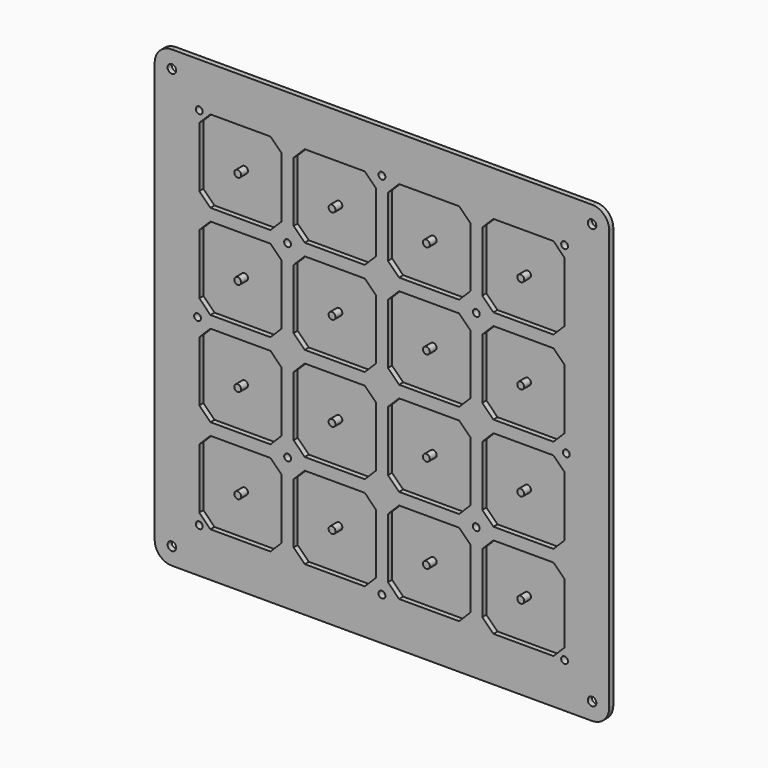
from build123d import *

# Parameters (mm, degrees)
F1_DEPTH      = 12
F2_START      = -12
F0_R          = 2
F2_DEPTH      = 6
F3_DEPTH      = 6
F4_DEPTH      = 20
F4_DEPTH_BACK = 5
F5_R          = 2.5
F6_DEPTH      = 3
F7_SIZE       = 2
F8_D          = 4
F8_2_D        = 4
F9_D          = 4


with BuildPart() as f1:
    # F0 (on Front) → F1 (new body)
    with BuildSketch(Plane.XZ):
        with BuildLine():
            Line((106.5, 111.5), (-106.5, 111.5))
            ThreePointArc((-106.5, 111.5), (-110.0355339059, 110.0355339059), (-111.5, 106.5))
            Line((-111.5, 106.5), (-111.5, -106.5))
            ThreePointArc((-111.5, -106.5), (-110.0355339059, -110.0355339059), (-106.5, -111.5))
            Line((-106.5, -111.5), (106.5, -111.5))
            ThreePointArc((106.5, -111.5), (110.0355339059, -110.0355339059), (111.5, -106.5))
            Line((111.5, -106.5), (111.5, 106.5))
            ThreePointArc((111.5, 106.5), (110.0355339059, 110.0355339059), (106.5, 111.5))
        make_face()
        Polygon((-64.5710678119, -57.5), (-57.5, -64.5710678119), (-57.5, -82.5), (-57.5, -100.4289321881), (-64.5710678119, -107.5), (-82.5, -107.5), (-100.4289321881, -107.5), (-107.5, -100.4289321881), (-107.5, -82.5), (-107.5, -64.5710678119), (-100.4289321881, -57.5), (-82.5, -57.5), align=None, mode=Mode.SUBTRACT)
        Polygon((-9.5710678119, -57.5), (-2.5, -64.5710678119), (-2.5, -82.5), (-2.5, -100.4289321881), (-9.5710678119, -107.5), (-27.5, -107.5), (-45.4289321881, -107.5), (-52.5, -100.4289321881), (-52.5, -82.5), (-52.5, -64.5710678119), (-45.4289321881, -57.5), (-27.5, -57.5), align=None, mode=Mode.SUBTRACT)
        Polygon((-64.5710678119, -2.5), (-57.5, -9.5710678119), (-57.5, -27.5), (-57.5, -45.4289321881), (-64.5710678119, -52.5), (-82.5, -52.5), (-100.4289321881, -52.5), (-107.5, -45.4289321881), (-107.5, -27.5), (-107.5, -9.5710678119), (-100.4289321881, -2.5), (-82.5, -2.5), align=None, mode=Mode.SUBTRACT)
        Polygon((-9.5710678119, -2.5), (-2.5, -9.5710678119), (-2.5, -27.5), (-2.5, -45.4289321881), (-9.5710678119, -52.5), (-27.5, -52.5), (-45.4289321881, -52.5), (-52.5, -45.4289321881), (-52.5, -27.5), (-52.5, -9.5710678119), (-45.4289321881, -2.5), (-27.5, -2.5), align=None, mode=Mode.SUBTRACT)
        Polygon((45.4289321881, -57.5), (52.5, -64.5710678119), (52.5, -82.5), (52.5, -100.4289321881), (45.4289321881, -107.5), (27.5, -107.5), (9.5710678119, -107.5), (2.5, -100.4289321881), (2.5, -82.5), (2.5, -64.5710678119), (9.5710678119, -57.5), (27.5, -57.5), align=None, mode=Mode.SUBTRACT)
        Polygon((100.4289321881, -57.5), (107.5, -64.5710678119), (107.5, -82.5), (107.5, -100.4289321881), (100.4289321881, -107.5), (82.5, -107.5), (64.5710678119, -107.5), (57.5, -100.4289321881), (57.5, -82.5), (57.5, -64.5710678119), (64.5710678119, -57.5), (82.5, -57.5), align=None, mode=Mode.SUBTRACT)
        Polygon((45.4289321881, -2.5), (52.5, -9.5710678119), (52.5, -27.5), (52.5, -45.4289321881), (45.4289321881, -52.5), (27.5, -52.5), (9.5710678119, -52.5), (2.5, -45.4289321881), (2.5, -27.5), (2.5, -9.5710678119), (9.5710678119, -2.5), (27.5, -2.5), align=None, mode=Mode.SUBTRACT)
        Polygon((100.4289321881, -2.5), (107.5, -9.5710678119), (107.5, -27.5), (107.5, -45.4289321881), (100.4289321881, -52.5), (82.5, -52.5), (64.5710678119, -52.5), (57.5, -45.4289321881), (57.5, -27.5), (57.5, -9.5710678119), (64.5710678119, -2.5), (82.5, -2.5), align=None, mode=Mode.SUBTRACT)
        Polygon((-64.5710678119, 52.5), (-57.5, 45.4289321881), (-57.5, 27.5), (-57.5, 9.5710678119), (-64.5710678119, 2.5), (-82.5, 2.5), (-100.4289321881, 2.5), (-107.5, 9.5710678119), (-107.5, 27.5), (-107.5, 45.4289321881), (-100.4289321881, 52.5), (-82.5, 52.5), align=None, mode=Mode.SUBTRACT)
        Polygon((-9.5710678119, 52.5), (-2.5, 45.4289321881), (-2.5, 27.5), (-2.5, 9.5710678119), (-9.5710678119, 2.5), (-27.5, 2.5), (-45.4289321881, 2.5), (-52.5, 9.5710678119), (-52.5, 27.5), (-52.5, 45.4289321881), (-45.4289321881, 52.5), (-27.5, 52.5), align=None, mode=Mode.SUBTRACT)
        Polygon((-107.5, 64.5710678119), (-107.5, 82.5), (-107.5, 100.4289321881), (-100.4289321881, 107.5), (-82.5, 107.5), (-64.5710678119, 107.5), (-57.5, 100.4289321881), (-57.5, 82.5), (-57.5, 64.5710678119), (-64.5710678119, 57.5), (-82.5, 57.5), (-100.4289321881, 57.5), align=None, mode=Mode.SUBTRACT)
        Polygon((-9.5710678119, 107.5), (-2.5, 100.4289321881), (-2.5, 82.5), (-2.5, 64.5710678119), (-9.5710678119, 57.5), (-27.5, 57.5), (-45.4289321881, 57.5), (-52.5, 64.5710678119), (-52.5, 82.5), (-52.5, 100.4289321881), (-45.4289321881, 107.5), (-27.5, 107.5), align=None, mode=Mode.SUBTRACT)
        Polygon((45.4289321881, 52.5), (52.5, 45.4289321881), (52.5, 27.5), (52.5, 9.5710678119), (45.4289321881, 2.5), (27.5, 2.5), (9.5710678119, 2.5), (2.5, 9.5710678119), (2.5, 27.5), (2.5, 45.4289321881), (9.5710678119, 52.5), (27.5, 52.5), align=None, mode=Mode.SUBTRACT)
        Polygon((100.4289321881, 52.5), (107.5, 45.4289321881), (107.5, 27.5), (107.5, 9.5710678119), (100.4289321881, 2.5), (82.5, 2.5), (64.5710678119, 2.5), (57.5, 9.5710678119), (57.5, 27.5), (57.5, 45.4289321881), (64.5710678119, 52.5), (82.5, 52.5), align=None, mode=Mode.SUBTRACT)
        Polygon((45.4289321881, 107.5), (52.5, 100.4289321881), (52.5, 82.5), (52.5, 64.5710678119), (45.4289321881, 57.5), (27.5, 57.5), (9.5710678119, 57.5), (2.5, 64.5710678119), (2.5, 82.5), (2.5, 100.4289321881), (9.5710678119, 107.5), (27.5, 107.5), align=None, mode=Mode.SUBTRACT)
        Polygon((100.4289321881, 107.5), (107.5, 100.4289321881), (107.5, 82.5), (107.5, 64.5710678119), (100.4289321881, 57.5), (82.5, 57.5), (64.5710678119, 57.5), (57.5, 64.5710678119), (57.5, 82.5), (57.5, 100.4289321881), (64.5710678119, 107.5), (82.5, 107.5), align=None, mode=Mode.SUBTRACT)
    extrude(amount=-F1_DEPTH)

    # F8 (through all)
    with Locations(Plane.XZ):
        with Locations((106.5, 106.5), (0, 107.5), (-106.5, 106.5), (-107.5, 0), (107.5, 0), (106.5, -106.5), (0, -107.5), (-106.5, -106.5), (-55, 55), (55, 55), (55, -55), (-55, -55)):
            Hole(F8_D / 2)


with BuildPart() as f2:
    # F0 (on Front) → F2 (new body)
    with BuildSketch(Plane.XZ.offset(F2_START)):
        with BuildLine():
            Line((106.5, 111.5), (-106.5, 111.5))
            ThreePointArc((-106.5, 111.5), (-110.0355339059, 110.0355339059), (-111.5, 106.5))
            Line((-111.5, 106.5), (-111.5, -106.5))
            ThreePointArc((-111.5, -106.5), (-110.0355339059, -110.0355339059), (-106.5, -111.5))
            Line((-106.5, -111.5), (106.5, -111.5))
            ThreePointArc((106.5, -111.5), (110.0355339059, -110.0355339059), (111.5, -106.5))
            Line((111.5, -106.5), (111.5, 106.5))
            ThreePointArc((111.5, 106.5), (110.0355339059, 110.0355339059), (106.5, 111.5))
        make_face()
        Polygon((-64.5710678119, -57.5), (-57.5, -64.5710678119), (-57.5, -82.5), (-57.5, -100.4289321881), (-64.5710678119, -107.5), (-82.5, -107.5), (-100.4289321881, -107.5), (-107.5, -100.4289321881), (-107.5, -82.5), (-107.5, -64.5710678119), (-100.4289321881, -57.5), (-82.5, -57.5), align=None, mode=Mode.SUBTRACT)
        Polygon((-9.5710678119, -57.5), (-2.5, -64.5710678119), (-2.5, -82.5), (-2.5, -100.4289321881), (-9.5710678119, -107.5), (-27.5, -107.5), (-45.4289321881, -107.5), (-52.5, -100.4289321881), (-52.5, -82.5), (-52.5, -64.5710678119), (-45.4289321881, -57.5), (-27.5, -57.5), align=None, mode=Mode.SUBTRACT)
        Polygon((-64.5710678119, -2.5), (-57.5, -9.5710678119), (-57.5, -27.5), (-57.5, -45.4289321881), (-64.5710678119, -52.5), (-82.5, -52.5), (-100.4289321881, -52.5), (-107.5, -45.4289321881), (-107.5, -27.5), (-107.5, -9.5710678119), (-100.4289321881, -2.5), (-82.5, -2.5), align=None, mode=Mode.SUBTRACT)
        Polygon((-9.5710678119, -2.5), (-2.5, -9.5710678119), (-2.5, -27.5), (-2.5, -45.4289321881), (-9.5710678119, -52.5), (-27.5, -52.5), (-45.4289321881, -52.5), (-52.5, -45.4289321881), (-52.5, -27.5), (-52.5, -9.5710678119), (-45.4289321881, -2.5), (-27.5, -2.5), align=None, mode=Mode.SUBTRACT)
        Polygon((45.4289321881, -57.5), (52.5, -64.5710678119), (52.5, -82.5), (52.5, -100.4289321881), (45.4289321881, -107.5), (27.5, -107.5), (9.5710678119, -107.5), (2.5, -100.4289321881), (2.5, -82.5), (2.5, -64.5710678119), (9.5710678119, -57.5), (27.5, -57.5), align=None, mode=Mode.SUBTRACT)
        Polygon((100.4289321881, -57.5), (107.5, -64.5710678119), (107.5, -82.5), (107.5, -100.4289321881), (100.4289321881, -107.5), (82.5, -107.5), (64.5710678119, -107.5), (57.5, -100.4289321881), (57.5, -82.5), (57.5, -64.5710678119), (64.5710678119, -57.5), (82.5, -57.5), align=None, mode=Mode.SUBTRACT)
        Polygon((45.4289321881, -2.5), (52.5, -9.5710678119), (52.5, -27.5), (52.5, -45.4289321881), (45.4289321881, -52.5), (27.5, -52.5), (9.5710678119, -52.5), (2.5, -45.4289321881), (2.5, -27.5), (2.5, -9.5710678119), (9.5710678119, -2.5), (27.5, -2.5), align=None, mode=Mode.SUBTRACT)
        Polygon((100.4289321881, -2.5), (107.5, -9.5710678119), (107.5, -27.5), (107.5, -45.4289321881), (100.4289321881, -52.5), (82.5, -52.5), (64.5710678119, -52.5), (57.5, -45.4289321881), (57.5, -27.5), (57.5, -9.5710678119), (64.5710678119, -2.5), (82.5, -2.5), align=None, mode=Mode.SUBTRACT)
        Polygon((-64.5710678119, 52.5), (-57.5, 45.4289321881), (-57.5, 27.5), (-57.5, 9.5710678119), (-64.5710678119, 2.5), (-82.5, 2.5), (-100.4289321881, 2.5), (-107.5, 9.5710678119), (-107.5, 27.5), (-107.5, 45.4289321881), (-100.4289321881, 52.5), (-82.5, 52.5), align=None, mode=Mode.SUBTRACT)
        Polygon((-9.5710678119, 52.5), (-2.5, 45.4289321881), (-2.5, 27.5), (-2.5, 9.5710678119), (-9.5710678119, 2.5), (-27.5, 2.5), (-45.4289321881, 2.5), (-52.5, 9.5710678119), (-52.5, 27.5), (-52.5, 45.4289321881), (-45.4289321881, 52.5), (-27.5, 52.5), align=None, mode=Mode.SUBTRACT)
        Polygon((-107.5, 64.5710678119), (-107.5, 82.5), (-107.5, 100.4289321881), (-100.4289321881, 107.5), (-82.5, 107.5), (-64.5710678119, 107.5), (-57.5, 100.4289321881), (-57.5, 82.5), (-57.5, 64.5710678119), (-64.5710678119, 57.5), (-82.5, 57.5), (-100.4289321881, 57.5), align=None, mode=Mode.SUBTRACT)
        Polygon((-9.5710678119, 107.5), (-2.5, 100.4289321881), (-2.5, 82.5), (-2.5, 64.5710678119), (-9.5710678119, 57.5), (-27.5, 57.5), (-45.4289321881, 57.5), (-52.5, 64.5710678119), (-52.5, 82.5), (-52.5, 100.4289321881), (-45.4289321881, 107.5), (-27.5, 107.5), align=None, mode=Mode.SUBTRACT)
        Polygon((45.4289321881, 52.5), (52.5, 45.4289321881), (52.5, 27.5), (52.5, 9.5710678119), (45.4289321881, 2.5), (27.5, 2.5), (9.5710678119, 2.5), (2.5, 9.5710678119), (2.5, 27.5), (2.5, 45.4289321881), (9.5710678119, 52.5), (27.5, 52.5), align=None, mode=Mode.SUBTRACT)
        Polygon((100.4289321881, 52.5), (107.5, 45.4289321881), (107.5, 27.5), (107.5, 9.5710678119), (100.4289321881, 2.5), (82.5, 2.5), (64.5710678119, 2.5), (57.5, 9.5710678119), (57.5, 27.5), (57.5, 45.4289321881), (64.5710678119, 52.5), (82.5, 52.5), align=None, mode=Mode.SUBTRACT)
        Polygon((45.4289321881, 107.5), (52.5, 100.4289321881), (52.5, 82.5), (52.5, 64.5710678119), (45.4289321881, 57.5), (27.5, 57.5), (9.5710678119, 57.5), (2.5, 64.5710678119), (2.5, 82.5), (2.5, 100.4289321881), (9.5710678119, 107.5), (27.5, 107.5), align=None, mode=Mode.SUBTRACT)
        Polygon((100.4289321881, 107.5), (107.5, 100.4289321881), (107.5, 82.5), (107.5, 64.5710678119), (100.4289321881, 57.5), (82.5, 57.5), (64.5710678119, 57.5), (57.5, 64.5710678119), (57.5, 82.5), (57.5, 100.4289321881), (64.5710678119, 107.5), (82.5, 107.5), align=None, mode=Mode.SUBTRACT)
        Polygon((107.5, -82.5), (107.5, -64.5710678119), (100.4289321881, -57.5), (82.5, -57.5), (64.5710678119, -57.5), (57.5, -64.5710678119), (57.5, -82.5), (57.5, -100.4289321881), (64.5710678119, -107.5), (82.5, -107.5), (100.4289321881, -107.5), (107.5, -100.4289321881), align=None)
        with Locations((82.5, -82.5)):
            Circle(F0_R, mode=Mode.SUBTRACT)
        Polygon((52.5, -82.5), (52.5, -64.5710678119), (45.4289321881, -57.5), (27.5, -57.5), (9.5710678119, -57.5), (2.5, -64.5710678119), (2.5, -82.5), (2.5, -100.4289321881), (9.5710678119, -107.5), (27.5, -107.5), (45.4289321881, -107.5), (52.5, -100.4289321881), align=None)
        with Locations((27.5, -82.5)):
            Circle(F0_R, mode=Mode.SUBTRACT)
        Polygon((-2.5, -82.5), (-2.5, -64.5710678119), (-9.5710678119, -57.5), (-27.5, -57.5), (-45.4289321881, -57.5), (-52.5, -64.5710678119), (-52.5, -82.5), (-52.5, -100.4289321881), (-45.4289321881, -107.5), (-27.5, -107.5), (-9.5710678119, -107.5), (-2.5, -100.4289321881), align=None)
        with Locations((-27.5, -82.5)):
            Circle(F0_R, mode=Mode.SUBTRACT)
        Polygon((-57.5, -82.5), (-57.5, -64.5710678119), (-64.5710678119, -57.5), (-82.5, -57.5), (-100.4289321881, -57.5), (-107.5, -64.5710678119), (-107.5, -82.5), (-107.5, -100.4289321881), (-100.4289321881, -107.5), (-82.5, -107.5), (-64.5710678119, -107.5), (-57.5, -100.4289321881), align=None)
        with Locations((-82.5, -82.5)):
            Circle(F0_R, mode=Mode.SUBTRACT)
        Polygon((-2.5, -27.5), (-2.5, -9.5710678119), (-9.5710678119, -2.5), (-27.5, -2.5), (-45.4289321881, -2.5), (-52.5, -9.5710678119), (-52.5, -27.5), (-52.5, -45.4289321881), (-45.4289321881, -52.5), (-27.5, -52.5), (-9.5710678119, -52.5), (-2.5, -45.4289321881), align=None)
        with Locations((-27.5, -27.5)):
            Circle(F0_R, mode=Mode.SUBTRACT)
        Polygon((-57.5, -27.5), (-57.5, -9.5710678119), (-64.5710678119, -2.5), (-82.5, -2.5), (-100.4289321881, -2.5), (-107.5, -9.5710678119), (-107.5, -27.5), (-107.5, -45.4289321881), (-100.4289321881, -52.5), (-82.5, -52.5), (-64.5710678119, -52.5), (-57.5, -45.4289321881), align=None)
        with Locations((-82.5, -27.5)):
            Circle(F0_R, mode=Mode.SUBTRACT)
        Polygon((52.5, -27.5), (52.5, -9.5710678119), (45.4289321881, -2.5), (27.5, -2.5), (9.5710678119, -2.5), (2.5, -9.5710678119), (2.5, -27.5), (2.5, -45.4289321881), (9.5710678119, -52.5), (27.5, -52.5), (45.4289321881, -52.5), (52.5, -45.4289321881), align=None)
        with Locations((27.5, -27.5)):
            Circle(F0_R, mode=Mode.SUBTRACT)
        Polygon((107.5, -27.5), (107.5, -9.5710678119), (100.4289321881, -2.5), (82.5, -2.5), (64.5710678119, -2.5), (57.5, -9.5710678119), (57.5, -27.5), (57.5, -45.4289321881), (64.5710678119, -52.5), (82.5, -52.5), (100.4289321881, -52.5), (107.5, -45.4289321881), align=None)
        with Locations((82.5, -27.5)):
            Circle(F0_R, mode=Mode.SUBTRACT)
        Polygon((107.5, 27.5), (107.5, 45.4289321881), (100.4289321881, 52.5), (82.5, 52.5), (64.5710678119, 52.5), (57.5, 45.4289321881), (57.5, 27.5), (57.5, 9.5710678119), (64.5710678119, 2.5), (82.5, 2.5), (100.4289321881, 2.5), (107.5, 9.5710678119), align=None)
        with Locations((82.5, 27.5)):
            Circle(F0_R, mode=Mode.SUBTRACT)
        Polygon((52.5, 27.5), (52.5, 45.4289321881), (45.4289321881, 52.5), (27.5, 52.5), (9.5710678119, 52.5), (2.5, 45.4289321881), (2.5, 27.5), (2.5, 9.5710678119), (9.5710678119, 2.5), (27.5, 2.5), (45.4289321881, 2.5), (52.5, 9.5710678119), align=None)
        with Locations((27.5, 27.5)):
            Circle(F0_R, mode=Mode.SUBTRACT)
        Polygon((-2.5, 27.5), (-2.5, 45.4289321881), (-9.5710678119, 52.5), (-27.5, 52.5), (-45.4289321881, 52.5), (-52.5, 45.4289321881), (-52.5, 27.5), (-52.5, 9.5710678119), (-45.4289321881, 2.5), (-27.5, 2.5), (-9.5710678119, 2.5), (-2.5, 9.5710678119), align=None)
        with Locations((-27.5, 27.5)):
            Circle(F0_R, mode=Mode.SUBTRACT)
        Polygon((-57.5, 27.5), (-57.5, 45.4289321881), (-64.5710678119, 52.5), (-82.5, 52.5), (-100.4289321881, 52.5), (-107.5, 45.4289321881), (-107.5, 27.5), (-107.5, 9.5710678119), (-100.4289321881, 2.5), (-82.5, 2.5), (-64.5710678119, 2.5), (-57.5, 9.5710678119), align=None)
        with Locations((-82.5, 27.5)):
            Circle(F0_R, mode=Mode.SUBTRACT)
        Polygon((-107.5, 100.4289321881), (-107.5, 82.5), (-107.5, 64.5710678119), (-100.4289321881, 57.5), (-82.5, 57.5), (-64.5710678119, 57.5), (-57.5, 64.5710678119), (-57.5, 82.5), (-57.5, 100.4289321881), (-64.5710678119, 107.5), (-82.5, 107.5), (-100.4289321881, 107.5), align=None)
        with Locations((-82.5, 82.5)):
            Circle(F0_R, mode=Mode.SUBTRACT)
        Polygon((-2.5, 82.5), (-2.5, 100.4289321881), (-9.5710678119, 107.5), (-27.5, 107.5), (-45.4289321881, 107.5), (-52.5, 100.4289321881), (-52.5, 82.5), (-52.5, 64.5710678119), (-45.4289321881, 57.5), (-27.5, 57.5), (-9.5710678119, 57.5), (-2.5, 64.5710678119), align=None)
        with Locations((-27.5, 82.5)):
            Circle(F0_R, mode=Mode.SUBTRACT)
        Polygon((52.5, 82.5), (52.5, 100.4289321881), (45.4289321881, 107.5), (27.5, 107.5), (9.5710678119, 107.5), (2.5, 100.4289321881), (2.5, 82.5), (2.5, 64.5710678119), (9.5710678119, 57.5), (27.5, 57.5), (45.4289321881, 57.5), (52.5, 64.5710678119), align=None)
        with Locations((27.5, 82.5)):
            Circle(F0_R, mode=Mode.SUBTRACT)
        Polygon((107.5, 82.5), (107.5, 100.4289321881), (100.4289321881, 107.5), (82.5, 107.5), (64.5710678119, 107.5), (57.5, 100.4289321881), (57.5, 82.5), (57.5, 64.5710678119), (64.5710678119, 57.5), (82.5, 57.5), (100.4289321881, 57.5), (107.5, 64.5710678119), align=None)
        with Locations((82.5, 82.5)):
            Circle(F0_R, mode=Mode.SUBTRACT)
    extrude(amount=-F2_DEPTH)

    # F7
    f7_edges = [f2.edges().sort_by_distance(p)[0] for p in [
        (-84.5, 12, 82.5),
        (-29.5, 12, 82.5),
        (25.5, 12, 82.5),
        (80.5, 12, 82.5),
        (80.5, 12, 27.5),
        (25.5, 12, 27.5),
        (-29.5, 12, 27.5),
        (-84.5, 12, 27.5),
        (-84.5, 12, -27.5),
        (-29.5, 12, -27.5),
        (25.5, 12, -27.5),
        (80.5, 12, -27.5),
        (80.5, 12, -82.5),
        (25.5, 12, -82.5),
        (-29.5, 12, -82.5),
        (-84.5, 12, -82.5),
    ]]
    chamfer(f7_edges, length=F7_SIZE)

    # F8#2 (through all)
    with Locations(Plane.XZ):
        with Locations((106.5, 106.5), (0, 107.5), (-106.5, 106.5), (-107.5, 0), (107.5, 0), (106.5, -106.5), (0, -107.5), (-106.5, -106.5), (-55, 55), (55, 55), (55, -55), (-55, -55)):
            Hole(F8_2_D / 2)


with BuildPart() as f3:
    # F0 (on Front) → F3 (new body)
    with BuildSketch(Plane.XZ):
        Polygon((-107.5, 100.4289321881), (-107.5, 82.5), (-107.5, 64.5710678119), (-100.4289321881, 57.5), (-82.5, 57.5), (-64.5710678119, 57.5), (-57.5, 64.5710678119), (-57.5, 82.5), (-57.5, 100.4289321881), (-64.5710678119, 107.5), (-82.5, 107.5), (-100.4289321881, 107.5), align=None)
        with Locations((-82.5, 82.5)):
            Circle(F0_R, mode=Mode.SUBTRACT)
    extrude(amount=-F3_DEPTH)


with BuildPart() as f3b:
    # F0 (on Front) → F3, piece 2 (new body)
    with BuildSketch(Plane.XZ):
        Polygon((-2.5, 82.5), (-2.5, 100.4289321881), (-9.5710678119, 107.5), (-27.5, 107.5), (-45.4289321881, 107.5), (-52.5, 100.4289321881), (-52.5, 82.5), (-52.5, 64.5710678119), (-45.4289321881, 57.5), (-27.5, 57.5), (-9.5710678119, 57.5), (-2.5, 64.5710678119), align=None)
        with Locations((-27.5, 82.5)):
            Circle(F0_R, mode=Mode.SUBTRACT)
    extrude(amount=-F3_DEPTH)


with BuildPart() as f3c:
    # F0 (on Front) → F3, piece 3 (new body)
    with BuildSketch(Plane.XZ):
        Polygon((52.5, 82.5), (52.5, 100.4289321881), (45.4289321881, 107.5), (27.5, 107.5), (9.5710678119, 107.5), (2.5, 100.4289321881), (2.5, 82.5), (2.5, 64.5710678119), (9.5710678119, 57.5), (27.5, 57.5), (45.4289321881, 57.5), (52.5, 64.5710678119), align=None)
        with Locations((27.5, 82.5)):
            Circle(F0_R, mode=Mode.SUBTRACT)
    extrude(amount=-F3_DEPTH)


with BuildPart() as f3d:
    # F0 (on Front) → F3, piece 4 (new body)
    with BuildSketch(Plane.XZ):
        Polygon((107.5, 82.5), (107.5, 100.4289321881), (100.4289321881, 107.5), (82.5, 107.5), (64.5710678119, 107.5), (57.5, 100.4289321881), (57.5, 82.5), (57.5, 64.5710678119), (64.5710678119, 57.5), (82.5, 57.5), (100.4289321881, 57.5), (107.5, 64.5710678119), align=None)
        with Locations((82.5, 82.5)):
            Circle(F0_R, mode=Mode.SUBTRACT)
    extrude(amount=-F3_DEPTH)


with BuildPart() as f3e:
    # F0 (on Front) → F3, piece 5 (new body)
    with BuildSketch(Plane.XZ):
        Polygon((-57.5, 27.5), (-57.5, 45.4289321881), (-64.5710678119, 52.5), (-82.5, 52.5), (-100.4289321881, 52.5), (-107.5, 45.4289321881), (-107.5, 27.5), (-107.5, 9.5710678119), (-100.4289321881, 2.5), (-82.5, 2.5), (-64.5710678119, 2.5), (-57.5, 9.5710678119), align=None)
        with Locations((-82.5, 27.5)):
            Circle(F0_R, mode=Mode.SUBTRACT)
    extrude(amount=-F3_DEPTH)


with BuildPart() as f3f:
    # F0 (on Front) → F3, piece 6 (new body)
    with BuildSketch(Plane.XZ):
        Polygon((-2.5, 27.5), (-2.5, 45.4289321881), (-9.5710678119, 52.5), (-27.5, 52.5), (-45.4289321881, 52.5), (-52.5, 45.4289321881), (-52.5, 27.5), (-52.5, 9.5710678119), (-45.4289321881, 2.5), (-27.5, 2.5), (-9.5710678119, 2.5), (-2.5, 9.5710678119), align=None)
        with Locations((-27.5, 27.5)):
            Circle(F0_R, mode=Mode.SUBTRACT)
    extrude(amount=-F3_DEPTH)


with BuildPart() as f3g:
    # F0 (on Front) → F3, piece 7 (new body)
    with BuildSketch(Plane.XZ):
        Polygon((52.5, 27.5), (52.5, 45.4289321881), (45.4289321881, 52.5), (27.5, 52.5), (9.5710678119, 52.5), (2.5, 45.4289321881), (2.5, 27.5), (2.5, 9.5710678119), (9.5710678119, 2.5), (27.5, 2.5), (45.4289321881, 2.5), (52.5, 9.5710678119), align=None)
        with Locations((27.5, 27.5)):
            Circle(F0_R, mode=Mode.SUBTRACT)
    extrude(amount=-F3_DEPTH)


with BuildPart() as f3h:
    # F0 (on Front) → F3, piece 8 (new body)
    with BuildSketch(Plane.XZ):
        Polygon((107.5, 27.5), (107.5, 45.4289321881), (100.4289321881, 52.5), (82.5, 52.5), (64.5710678119, 52.5), (57.5, 45.4289321881), (57.5, 27.5), (57.5, 9.5710678119), (64.5710678119, 2.5), (82.5, 2.5), (100.4289321881, 2.5), (107.5, 9.5710678119), align=None)
        with Locations((82.5, 27.5)):
            Circle(F0_R, mode=Mode.SUBTRACT)
    extrude(amount=-F3_DEPTH)


with BuildPart() as f3i:
    # F0 (on Front) → F3, piece 9 (new body)
    with BuildSketch(Plane.XZ):
        Polygon((107.5, -27.5), (107.5, -9.5710678119), (100.4289321881, -2.5), (82.5, -2.5), (64.5710678119, -2.5), (57.5, -9.5710678119), (57.5, -27.5), (57.5, -45.4289321881), (64.5710678119, -52.5), (82.5, -52.5), (100.4289321881, -52.5), (107.5, -45.4289321881), align=None)
        with Locations((82.5, -27.5)):
            Circle(F0_R, mode=Mode.SUBTRACT)
    extrude(amount=-F3_DEPTH)


with BuildPart() as f3j:
    # F0 (on Front) → F3, piece 10 (new body)
    with BuildSketch(Plane.XZ):
        Polygon((52.5, -27.5), (52.5, -9.5710678119), (45.4289321881, -2.5), (27.5, -2.5), (9.5710678119, -2.5), (2.5, -9.5710678119), (2.5, -27.5), (2.5, -45.4289321881), (9.5710678119, -52.5), (27.5, -52.5), (45.4289321881, -52.5), (52.5, -45.4289321881), align=None)
        with Locations((27.5, -27.5)):
            Circle(F0_R, mode=Mode.SUBTRACT)
    extrude(amount=-F3_DEPTH)


with BuildPart() as f3k:
    # F0 (on Front) → F3, piece 11 (new body)
    with BuildSketch(Plane.XZ):
        Polygon((-2.5, -27.5), (-2.5, -9.5710678119), (-9.5710678119, -2.5), (-27.5, -2.5), (-45.4289321881, -2.5), (-52.5, -9.5710678119), (-52.5, -27.5), (-52.5, -45.4289321881), (-45.4289321881, -52.5), (-27.5, -52.5), (-9.5710678119, -52.5), (-2.5, -45.4289321881), align=None)
        with Locations((-27.5, -27.5)):
            Circle(F0_R, mode=Mode.SUBTRACT)
    extrude(amount=-F3_DEPTH)


with BuildPart() as f3l:
    # F0 (on Front) → F3, piece 12 (new body)
    with BuildSketch(Plane.XZ):
        Polygon((-57.5, -27.5), (-57.5, -9.5710678119), (-64.5710678119, -2.5), (-82.5, -2.5), (-100.4289321881, -2.5), (-107.5, -9.5710678119), (-107.5, -27.5), (-107.5, -45.4289321881), (-100.4289321881, -52.5), (-82.5, -52.5), (-64.5710678119, -52.5), (-57.5, -45.4289321881), align=None)
        with Locations((-82.5, -27.5)):
            Circle(F0_R, mode=Mode.SUBTRACT)
    extrude(amount=-F3_DEPTH)


with BuildPart() as f3m:
    # F0 (on Front) → F3, piece 13 (new body)
    with BuildSketch(Plane.XZ):
        Polygon((-57.5, -82.5), (-57.5, -64.5710678119), (-64.5710678119, -57.5), (-82.5, -57.5), (-100.4289321881, -57.5), (-107.5, -64.5710678119), (-107.5, -82.5), (-107.5, -100.4289321881), (-100.4289321881, -107.5), (-82.5, -107.5), (-64.5710678119, -107.5), (-57.5, -100.4289321881), align=None)
        with Locations((-82.5, -82.5)):
            Circle(F0_R, mode=Mode.SUBTRACT)
    extrude(amount=-F3_DEPTH)


with BuildPart() as f3n:
    # F0 (on Front) → F3, piece 14 (new body)
    with BuildSketch(Plane.XZ):
        Polygon((-2.5, -82.5), (-2.5, -64.5710678119), (-9.5710678119, -57.5), (-27.5, -57.5), (-45.4289321881, -57.5), (-52.5, -64.5710678119), (-52.5, -82.5), (-52.5, -100.4289321881), (-45.4289321881, -107.5), (-27.5, -107.5), (-9.5710678119, -107.5), (-2.5, -100.4289321881), align=None)
        with Locations((-27.5, -82.5)):
            Circle(F0_R, mode=Mode.SUBTRACT)
    extrude(amount=-F3_DEPTH)


with BuildPart() as f3o:
    # F0 (on Front) → F3, piece 15 (new body)
    with BuildSketch(Plane.XZ):
        Polygon((52.5, -82.5), (52.5, -64.5710678119), (45.4289321881, -57.5), (27.5, -57.5), (9.5710678119, -57.5), (2.5, -64.5710678119), (2.5, -82.5), (2.5, -100.4289321881), (9.5710678119, -107.5), (27.5, -107.5), (45.4289321881, -107.5), (52.5, -100.4289321881), align=None)
        with Locations((27.5, -82.5)):
            Circle(F0_R, mode=Mode.SUBTRACT)
    extrude(amount=-F3_DEPTH)


with BuildPart() as f3p:
    # F0 (on Front) → F3, piece 16 (new body)
    with BuildSketch(Plane.XZ):
        Polygon((107.5, -82.5), (107.5, -64.5710678119), (100.4289321881, -57.5), (82.5, -57.5), (64.5710678119, -57.5), (57.5, -64.5710678119), (57.5, -82.5), (57.5, -100.4289321881), (64.5710678119, -107.5), (82.5, -107.5), (100.4289321881, -107.5), (107.5, -100.4289321881), align=None)
        with Locations((82.5, -82.5)):
            Circle(F0_R, mode=Mode.SUBTRACT)
    extrude(amount=-F3_DEPTH)


with BuildPart() as f4:
    # F0 (on Front) → F4 (new body, two sides)
    with BuildSketch(Plane.XZ) as f4_sk:
        with Locations((-27.5, 82.5)):
            Circle(F0_R)
    extrude(amount=-F4_DEPTH)
    extrude(f4_sk.sketch, amount=F4_DEPTH_BACK)


with BuildPart() as f4b:
    # F0 (on Front) → F4, piece 2 (new body, two sides)
    with BuildSketch(Plane.XZ) as f4_2_sk:
        with Locations((27.5, 82.5)):
            Circle(F0_R)
    extrude(amount=-F4_DEPTH)
    extrude(f4_2_sk.sketch, amount=F4_DEPTH_BACK)


with BuildPart() as f4c:
    # F0 (on Front) → F4, piece 3 (new body, two sides)
    with BuildSketch(Plane.XZ) as f4_3_sk:
        with Locations((82.5, 82.5)):
            Circle(F0_R)
    extrude(amount=-F4_DEPTH)
    extrude(f4_3_sk.sketch, amount=F4_DEPTH_BACK)


with BuildPart() as f4d:
    # F0 (on Front) → F4, piece 4 (new body, two sides)
    with BuildSketch(Plane.XZ) as f4_4_sk:
        with Locations((-82.5, 27.5)):
            Circle(F0_R)
    extrude(amount=-F4_DEPTH)
    extrude(f4_4_sk.sketch, amount=F4_DEPTH_BACK)


with BuildPart() as f4e:
    # F0 (on Front) → F4, piece 5 (new body, two sides)
    with BuildSketch(Plane.XZ) as f4_5_sk:
        with Locations((-27.5, 27.5)):
            Circle(F0_R)
    extrude(amount=-F4_DEPTH)
    extrude(f4_5_sk.sketch, amount=F4_DEPTH_BACK)


with BuildPart() as f4f:
    # F0 (on Front) → F4, piece 6 (new body, two sides)
    with BuildSketch(Plane.XZ) as f4_6_sk:
        with Locations((27.5, 27.5)):
            Circle(F0_R)
    extrude(amount=-F4_DEPTH)
    extrude(f4_6_sk.sketch, amount=F4_DEPTH_BACK)


with BuildPart() as f4g:
    # F0 (on Front) → F4, piece 7 (new body, two sides)
    with BuildSketch(Plane.XZ) as f4_7_sk:
        with Locations((82.5, 27.5)):
            Circle(F0_R)
    extrude(amount=-F4_DEPTH)
    extrude(f4_7_sk.sketch, amount=F4_DEPTH_BACK)


with BuildPart() as f4h:
    # F0 (on Front) → F4, piece 8 (new body, two sides)
    with BuildSketch(Plane.XZ) as f4_8_sk:
        with Locations((-82.5, -27.5)):
            Circle(F0_R)
    extrude(amount=-F4_DEPTH)
    extrude(f4_8_sk.sketch, amount=F4_DEPTH_BACK)


with BuildPart() as f4i:
    # F0 (on Front) → F4, piece 9 (new body, two sides)
    with BuildSketch(Plane.XZ) as f4_9_sk:
        with Locations((-27.5, -27.5)):
            Circle(F0_R)
    extrude(amount=-F4_DEPTH)
    extrude(f4_9_sk.sketch, amount=F4_DEPTH_BACK)


with BuildPart() as f4j:
    # F0 (on Front) → F4, piece 10 (new body, two sides)
    with BuildSketch(Plane.XZ) as f4_10_sk:
        with Locations((27.5, -27.5)):
            Circle(F0_R)
    extrude(amount=-F4_DEPTH)
    extrude(f4_10_sk.sketch, amount=F4_DEPTH_BACK)


with BuildPart() as f4k:
    # F0 (on Front) → F4, piece 11 (new body, two sides)
    with BuildSketch(Plane.XZ) as f4_11_sk:
        with Locations((82.5, -27.5)):
            Circle(F0_R)
    extrude(amount=-F4_DEPTH)
    extrude(f4_11_sk.sketch, amount=F4_DEPTH_BACK)


with BuildPart() as f4l:
    # F0 (on Front) → F4, piece 12 (new body, two sides)
    with BuildSketch(Plane.XZ) as f4_12_sk:
        with Locations((-82.5, -82.5)):
            Circle(F0_R)
    extrude(amount=-F4_DEPTH)
    extrude(f4_12_sk.sketch, amount=F4_DEPTH_BACK)


with BuildPart() as f4m:
    # F0 (on Front) → F4, piece 13 (new body, two sides)
    with BuildSketch(Plane.XZ) as f4_13_sk:
        with Locations((-27.5, -82.5)):
            Circle(F0_R)
    extrude(amount=-F4_DEPTH)
    extrude(f4_13_sk.sketch, amount=F4_DEPTH_BACK)


with BuildPart() as f4n:
    # F0 (on Front) → F4, piece 14 (new body, two sides)
    with BuildSketch(Plane.XZ) as f4_14_sk:
        with Locations((27.5, -82.5)):
            Circle(F0_R)
    extrude(amount=-F4_DEPTH)
    extrude(f4_14_sk.sketch, amount=F4_DEPTH_BACK)


with BuildPart() as f4o:
    # F0 (on Front) → F4, piece 15 (new body, two sides)
    with BuildSketch(Plane.XZ) as f4_15_sk:
        with Locations((82.5, -82.5)):
            Circle(F0_R)
    extrude(amount=-F4_DEPTH)
    extrude(f4_15_sk.sketch, amount=F4_DEPTH_BACK)


with BuildPart() as f4p:
    # F0 (on Front) → F4, piece 16 (new body, two sides)
    with BuildSketch(Plane.XZ) as f4_16_sk:
        with Locations((-82.5, 82.5)):
            Circle(F0_R)
    extrude(amount=-F4_DEPTH)
    extrude(f4_16_sk.sketch, amount=F4_DEPTH_BACK)


with BuildPart() as f6:
    # F5 (on face) → F6 (new body)
    with BuildSketch(Plane.XZ):
        with BuildLine():
            Line((122.5, 132.5), (-122.5, 132.5))
            ThreePointArc((-122.5, 132.5), (-129.5710678119, 129.5710678119), (-132.5, 122.5))
            Line((-132.5, 122.5), (-132.5, -122.5))
            ThreePointArc((-132.5, -122.5), (-129.5710678119, -129.5710678119), (-122.5, -132.5))
            Line((-122.5, -132.5), (122.5, -132.5))
            ThreePointArc((122.5, -132.5), (129.5710678119, -129.5710678119), (132.5, -122.5))
            Line((132.5, -122.5), (132.5, 122.5))
            ThreePointArc((132.5, 122.5), (129.5710678119, 129.5710678119), (122.5, 132.5))
        make_face()
        with Locations((-122.5, -122.5)):
            Circle(F5_R, mode=Mode.SUBTRACT)
        Polygon((-58.5, -100.0147186258), (-64.9852813742, -106.5), (-100.0147186258, -106.5), (-106.5, -100.0147186258), (-106.5, -64.9852813742), (-100.0147186258, -58.5), (-64.9852813742, -58.5), (-58.5, -64.9852813742), align=None, mode=Mode.SUBTRACT)
        Polygon((-3.5, -100.0147186258), (-9.9852813742, -106.5), (-45.0147186258, -106.5), (-51.5, -100.0147186258), (-51.5, -64.9852813742), (-45.0147186258, -58.5), (-9.9852813742, -58.5), (-3.5, -64.9852813742), align=None, mode=Mode.SUBTRACT)
        Polygon((-58.5, -45.0147186258), (-64.9852813742, -51.5), (-100.0147186258, -51.5), (-106.5, -45.0147186258), (-106.5, -9.9852813742), (-100.0147186258, -3.5), (-64.9852813742, -3.5), (-58.5, -9.9852813742), align=None, mode=Mode.SUBTRACT)
        Polygon((-3.5, -45.0147186258), (-9.9852813742, -51.5), (-45.0147186258, -51.5), (-51.5, -45.0147186258), (-51.5, -9.9852813742), (-45.0147186258, -3.5), (-9.9852813742, -3.5), (-3.5, -9.9852813742), align=None, mode=Mode.SUBTRACT)
        Polygon((51.5, -100.0147186258), (45.0147186258, -106.5), (9.9852813742, -106.5), (3.5, -100.0147186258), (3.5, -64.9852813742), (9.9852813742, -58.5), (45.0147186258, -58.5), (51.5, -64.9852813742), align=None, mode=Mode.SUBTRACT)
        with Locations((122.5, -122.5)):
            Circle(F5_R, mode=Mode.SUBTRACT)
        Polygon((106.5, -100.0147186258), (100.0147186258, -106.5), (64.9852813742, -106.5), (58.5, -100.0147186258), (58.5, -64.9852813742), (64.9852813742, -58.5), (100.0147186258, -58.5), (106.5, -64.9852813742), align=None, mode=Mode.SUBTRACT)
        Polygon((51.5, -45.0147186258), (45.0147186258, -51.5), (9.9852813742, -51.5), (3.5, -45.0147186258), (3.5, -9.9852813742), (9.9852813742, -3.5), (45.0147186258, -3.5), (51.5, -9.9852813742), align=None, mode=Mode.SUBTRACT)
        Polygon((106.5, -45.0147186258), (100.0147186258, -51.5), (64.9852813742, -51.5), (58.5, -45.0147186258), (58.5, -9.9852813742), (64.9852813742, -3.5), (100.0147186258, -3.5), (106.5, -9.9852813742), align=None, mode=Mode.SUBTRACT)
        Polygon((-58.5, 9.9852813742), (-64.9852813742, 3.5), (-100.0147186258, 3.5), (-106.5, 9.9852813742), (-106.5, 45.0147186258), (-100.0147186258, 51.5), (-64.9852813742, 51.5), (-58.5, 45.0147186258), align=None, mode=Mode.SUBTRACT)
        Polygon((-3.5, 9.9852813742), (-9.9852813742, 3.5), (-45.0147186258, 3.5), (-51.5, 9.9852813742), (-51.5, 45.0147186258), (-45.0147186258, 51.5), (-9.9852813742, 51.5), (-3.5, 45.0147186258), align=None, mode=Mode.SUBTRACT)
        Polygon((-106.5, 100.0147186258), (-100.0147186258, 106.5), (-64.9852813742, 106.5), (-58.5, 100.0147186258), (-58.5, 64.9852813742), (-64.9852813742, 58.5), (-100.0147186258, 58.5), (-106.5, 64.9852813742), align=None, mode=Mode.SUBTRACT)
        with Locations((-122.5, 122.5)):
            Circle(F5_R, mode=Mode.SUBTRACT)
        Polygon((-3.5, 64.9852813742), (-9.9852813742, 58.5), (-45.0147186258, 58.5), (-51.5, 64.9852813742), (-51.5, 100.0147186258), (-45.0147186258, 106.5), (-9.9852813742, 106.5), (-3.5, 100.0147186258), align=None, mode=Mode.SUBTRACT)
        Polygon((51.5, 9.9852813742), (45.0147186258, 3.5), (9.9852813742, 3.5), (3.5, 9.9852813742), (3.5, 45.0147186258), (9.9852813742, 51.5), (45.0147186258, 51.5), (51.5, 45.0147186258), align=None, mode=Mode.SUBTRACT)
        Polygon((106.5, 9.9852813742), (100.0147186258, 3.5), (64.9852813742, 3.5), (58.5, 9.9852813742), (58.5, 45.0147186258), (64.9852813742, 51.5), (100.0147186258, 51.5), (106.5, 45.0147186258), align=None, mode=Mode.SUBTRACT)
        Polygon((51.5, 64.9852813742), (45.0147186258, 58.5), (9.9852813742, 58.5), (3.5, 64.9852813742), (3.5, 100.0147186258), (9.9852813742, 106.5), (45.0147186258, 106.5), (51.5, 100.0147186258), align=None, mode=Mode.SUBTRACT)
        Polygon((106.5, 64.9852813742), (100.0147186258, 58.5), (64.9852813742, 58.5), (58.5, 64.9852813742), (58.5, 100.0147186258), (64.9852813742, 106.5), (100.0147186258, 106.5), (106.5, 100.0147186258), align=None, mode=Mode.SUBTRACT)
        with Locations((122.5, 122.5)):
            Circle(F5_R, mode=Mode.SUBTRACT)
    extrude(amount=F6_DEPTH)

    # F9 (through all)
    with Locations(Plane(origin=(0, 0, 0), x_dir=(1, 0, 0), z_dir=(0, 1, 0))):
        with Locations((106.5, 106.5), (0, 107.5), (-106.5, 106.5), (-107.5, 0), (-55, 55), (55, 55), (107.5, 0), (55, -55), (-55, -55), (-106.5, -106.5), (0, -107.5), (106.5, -106.5)):
            Hole(F9_D / 2)


solid = Compound([f1.part, f2.part, f3.part, f3b.part, f3c.part, f3d.part, f3e.part, f3f.part, f3g.part, f3h.part, f3i.part, f3j.part, f3k.part, f3l.part, f3m.part, f3n.part, f3o.part, f3p.part, f4.part, f4b.part, f4c.part, f4d.part, f4e.part, f4f.part, f4g.part, f4h.part, f4i.part, f4j.part, f4k.part, f4l.part, f4m.part, f4n.part, f4o.part, f4p.part, f6.part])
